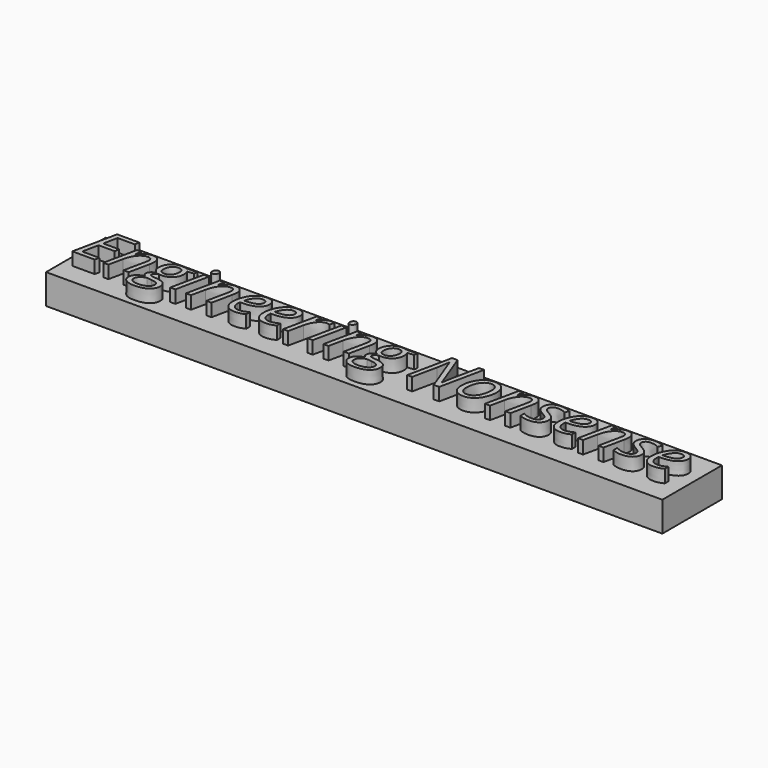
from build123d import *

# Parameters (mm, degrees)
F0_TEXT_SIZE = 14.5456906768
F1_DEPTH     = 10
F2_W         = 144.3562544882
F2_H         = 17.4496578984
F3_DEPTH     = 7


# Not quite as in the source:
# - Text() gives the source's letters only with a copy of the font that has no kerning and outlines rounded to 1/6400 em; it was checked with that copy


with BuildPart() as f1:
    # F0 (on Top) → F1 (new body)
    with BuildSketch(Plane.XY):
        with Locations((-15.6005290464, 0.4862318963)):
            Text('Engineering Nonsense', F0_TEXT_SIZE, font='Open Sans', font_style=FontStyle.ITALIC, text_align=(TextAlign.LEFT, TextAlign.BOTTOM))
    extrude(amount=F1_DEPTH)

    # F2 (on Top) → F3 (join)
    with BuildSketch(Plane.XY):
        with Locations((54.9718867987, 4.2943966109)):
            Rectangle(F2_W, F2_H)
    extrude(amount=F3_DEPTH)


solid = f1.part
